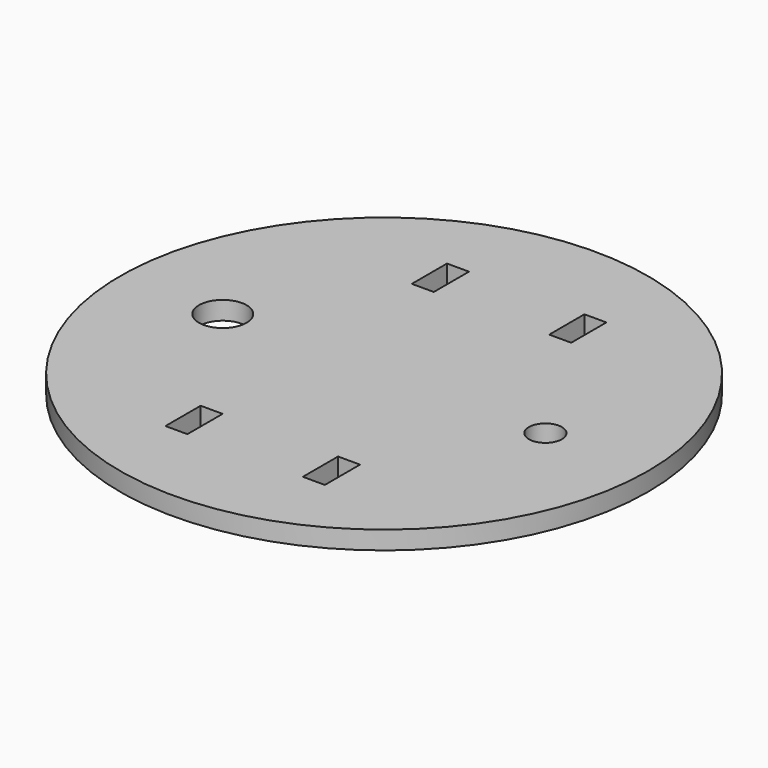
from build123d import *

# Parameters (mm, degrees)
F0_R     = 114.3
F0_W     = 9.525
F0_H     = 19.05
F0_R_2   = 10.31875
F0_R_3   = 7.14375
F1_DEPTH = 7.9375


# Not quite as in the source:
# - a length typed as a fraction of an inch, garbled in the dataset ("3 / 203.2 mm" for 3/8 in), is restored


with BuildPart() as f1:
    # F0 (on Top) → F1 (new body)
    with BuildSketch(Plane.XY):
        Circle(F0_R)
        with Locations((-28.9588448, -66.675)):
            Rectangle(F0_W, F0_H, mode=Mode.SUBTRACT)
        with Locations((30.5463448, -66.675)):
            Rectangle(F0_W, F0_H, mode=Mode.SUBTRACT)
        with Locations((-69.85, 0)):
            Circle(F0_R_2, mode=Mode.SUBTRACT)
        with Locations((-28.9588448, 66.675)):
            Rectangle(F0_W, F0_H, mode=Mode.SUBTRACT)
        with Locations((69.85, 0)):
            Circle(F0_R_3, mode=Mode.SUBTRACT)
        with Locations((30.5463448, 66.675)):
            Rectangle(F0_W, F0_H, mode=Mode.SUBTRACT)
    extrude(amount=F1_DEPTH)


solid = f1.part
